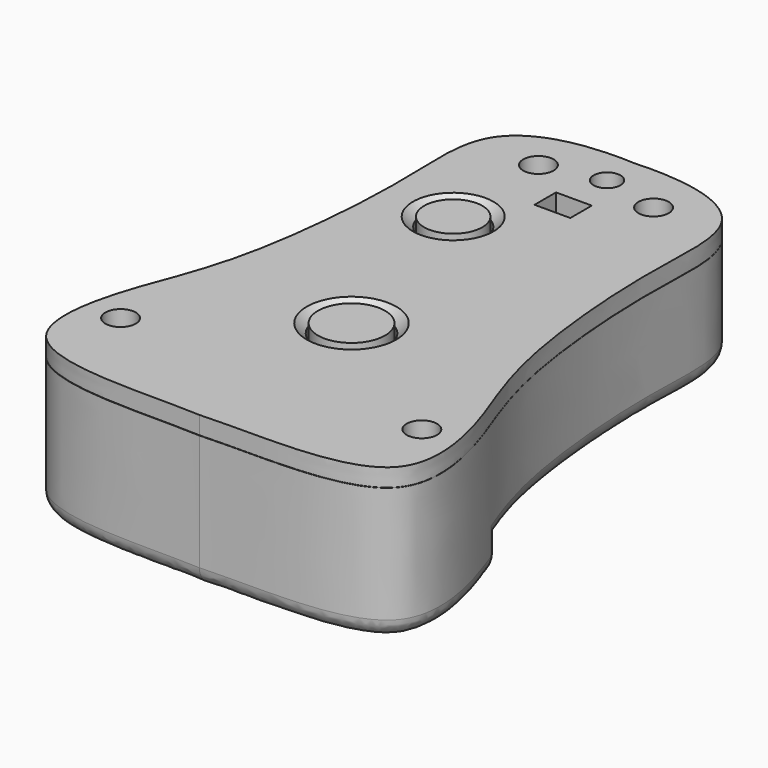
from build123d import *

# Parameters (mm, degrees)
F2_W          = 29
F2_H          = 13
F2_R          = 1.5
F3_DEPTH      = 15
F4_W          = 13.7690324336
F4_H          = 2.1893926171
F5_DEPTH      = 10
F6_DEPTH      = 13
F7_W          = 47.3588760942
F7_H          = 46.9052456319
F8_DEPTH      = 3
F8_DEPTH_BACK = 25
F10_R         = 4
F10_R_2       = 3.5
F10_W         = 4
F10_H         = 3
F10_R_3       = 1.5
F11_DEPTH     = 2
F12_R         = 3.25
F13_DEPTH     = 6
F12_R_2       = 3.75
F14_R         = 4.5
F16_DEPTH     = 2
F15_R         = 4
F17_SIZE      = 1
F18_R         = 2
F19_D         = 3.4
F19_2_D       = 3.4


# Not quite as in the source:
# - a feature names something its author has since deleted; it is built from what else it names


with BuildPart() as f3:
    # F2 (on Top) → F3 (new body)
    with BuildSketch(Plane.XY):
        with BuildLine():
            add(Edge.make_bspline(
                [(0, -18.8045408577), (-6.330118611, -18.4665963498), (-24.8841015024, -20.3961867477), (-19.1041639634, -2.5898293205), (-18.0902377672, -0.1629577332), (-15.4149948763, 7.458109725), (-13.9668437302, 19.9197467311), (-13.8469548104, 29.1685827727), (-14.5035852965, 40.0910711005), (-6.177108239, 42.3723793593), (0, 42.037602514)],
                knots=[0, 0, 0, 0, 0.1734330727, 0.310473001, 0.3791785419, 0.4845453033, 0.6233790216, 0.7442869454, 0.8592242244, 1, 1, 1, 1], degree=3))
            add(Edge.make_bspline(
                [(0, -18.8045408577), (6.330118611, -18.4665963498), (24.8841015024, -20.3961867477), (19.1041639634, -2.5898293205), (18.0902377672, -0.1629577332), (15.4149948763, 7.458109725), (13.9668437302, 19.9197467311), (13.8469548104, 29.1685827727), (14.5035852965, 40.0910711005), (6.177108239, 42.3723793593), (0, 42.037602514)],
                knots=[0, 0, 0, 0, 0.1734330727, 0.310473001, 0.3791785419, 0.4845453033, 0.6233790216, 0.7442869454, 0.8592242244, 1, 1, 1, 1], degree=3))
        make_face()
        with Locations((0, -8.6893926171)):
            Rectangle(F2_W, F2_H, mode=Mode.SUBTRACT)
        with Locations((0, 38.0456671119)):
            Circle(F2_R, mode=Mode.SUBTRACT)
        with Locations((0, -8.6893926171)):
            Rectangle(F2_W, F2_H)
    extrude(amount=F3_DEPTH)

    # F4 (on face) → F5 (cut)
    with BuildSketch(Plane.XY.offset(15)):
        Polygon((10.7, 33.9), (-10.7, 33.9), (-10.7, 0), (-6.8845162168, 0), (6.8845162168, 0), (10.7, 0), align=None)
        with Locations((0, -1.0946963086)):
            Rectangle(F4_W, F4_H)
    extrude(amount=-F5_DEPTH, mode=Mode.SUBTRACT)

    # F4 (on face) → F6 (cut)
    with BuildSketch(Plane.XY.offset(15)):
        Polygon((6.8845162168, -2.1893926171), (-6.8845162168, -2.1893926171), (-14.5, -2.1893926171), (-14.5, -15.1893926171), (14.5, -15.1893926171), (14.5, -2.1893926171), align=None)
    extrude(amount=-F6_DEPTH, mode=Mode.SUBTRACT)

    # F7 (on Top) → F8 (cut, two sides)
    with BuildSketch(Plane.XY) as f8_sk:
        with Locations((-0.3629019484, 23.452622816)):
            Rectangle(F7_W, F7_H)
    extrude(amount=F8_DEPTH, mode=Mode.SUBTRACT)
    extrude(f8_sk.sketch, amount=-F8_DEPTH_BACK, mode=Mode.SUBTRACT)

    # F18
    f18_edges = [f3.edges().sort_by_distance(p)[0] for p in [
        (13.931057, 25.9215, 3),
        (-13.931057, 25.9215, 3),
        (0, 0, 0),
        (-18.100143, -16.893942, 0),
        (18.100143, -16.893942, 0),
        (-18.066248, 0, 1.5),
        (18.066248, 0, 1.5),
    ]]
    fillet(f18_edges, radius=F18_R)

    # F19 (through all)
    with Locations(Plane(origin=(0, 0, 0), x_dir=(1, 0, 0), z_dir=(0, 0, -1))):
        with Locations((-16.8293025345, 8.7669137865), (16.8293025345, 8.7669137865), (6.4332578331, -36.594055593), (-6.4332578331, -36.594055593)):
            Hole(F19_D / 2)


with BuildPart() as f11:
    # F10 (on offset) → F11 (new body)
    with BuildSketch(Plane.XY.offset(15)):
        with BuildLine():
            add(Edge.make_bspline(
                [(-0.0276851933, -18.7595865615), (-6.3578038044, -18.4216420536), (-24.9117866957, -20.3512324514), (-19.1318491568, -2.5448750243), (-18.1179229605, -0.118003437), (-15.4426800696, 7.5030640212), (-13.9945289236, 19.9647010273), (-13.8746400037, 29.2135370689), (-14.5312704898, 40.1360253967), (-6.2047934323, 42.4173336555), (-0.0276851933, 42.0825568102)],
                knots=[0, 0, 0, 0, 0.1734330727, 0.310473001, 0.3791785419, 0.4845453033, 0.6233790216, 0.7442869454, 0.8592242244, 1, 1, 1, 1], degree=3))
            add(Edge.make_bspline(
                [(-0.0276851933, -18.7595865615), (6.3024334177, -18.4216420536), (24.856416309, -20.3512324514), (19.0764787701, -2.5448750243), (18.0625525738, -0.118003437), (15.3873096829, 7.5030640212), (13.9391585369, 19.9647010273), (13.819269617, 29.2135370689), (14.4759001031, 40.1360253967), (6.1494230457, 42.4173336555), (-0.0276851933, 42.0825568102)],
                knots=[0, 0, 0, 0, 0.1734330727, 0.310473001, 0.3791785419, 0.4845453033, 0.6233790216, 0.7442869454, 0.8592242244, 1, 1, 1, 1], degree=3))
        make_face()
        with Locations((-0.4992242519, 3.0747483215)):
            Circle(F10_R, mode=Mode.SUBTRACT)
        with Locations((-6.1522662348, 24.3455740829)):
            Circle(F10_R_2, mode=Mode.SUBTRACT)
        with Locations((0, 32.0099077523)):
            Rectangle(F10_W, F10_H, mode=Mode.SUBTRACT)
        with Locations((0.0476241112, 38.0757294449)):
            Circle(F10_R_3, mode=Mode.SUBTRACT)
    extrude(amount=F11_DEPTH)

    # F17
    f17_edges = [f11.edges().sort_by_distance(p)[0] for p in [
        (-9.652266, 24.345574, 17),
        (-4.499224, 3.074748, 17),
    ]]
    chamfer(f17_edges, length=F17_SIZE)

    # F19#2 (through all)
    with Locations(Plane(origin=(0, 0, 0), x_dir=(1, 0, 0), z_dir=(0, 0, -1))):
        with Locations((-16.8293025345, 8.7669137865), (16.8293025345, 8.7669137865), (6.4332578331, -36.594055593), (-6.4332578331, -36.594055593)):
            Hole(F19_2_D / 2)


with BuildPart() as f13:
    # F12 (on face) → F13 (new body)
    with BuildSketch(Plane.XY.offset(17)):
        with Locations((-6.1522662348, 24.3455740829)):
            Circle(F12_R)
    extrude(amount=-F13_DEPTH)

    # F15 (on face) → F16, piece 2 (join)
    with BuildSketch(Plane(origin=(0, 0, 11), x_dir=(1, 0, 0), z_dir=(0, 0, -1))):
        with Locations((-6.1522662348, -24.3455740829)):
            Circle(F15_R)
    extrude(amount=-F16_DEPTH)


with BuildPart() as f13b:
    # F12 (on face) → F13, piece 2 (new body)
    with BuildSketch(Plane.XY.offset(17)):
        with Locations((-0.4992242519, 3.0747483215)):
            Circle(F12_R_2)
    extrude(amount=-F13_DEPTH)

    # F14 (on face) → F16 (join)
    with BuildSketch(Plane(origin=(0, 0, 11), x_dir=(1, 0, 0), z_dir=(0, 0, -1))):
        with Locations((-0.4992242519, -3.0747483215)):
            Circle(F14_R)
    extrude(amount=-F16_DEPTH)


solid = Compound([f3.part, f11.part, f13.part, f13b.part])
